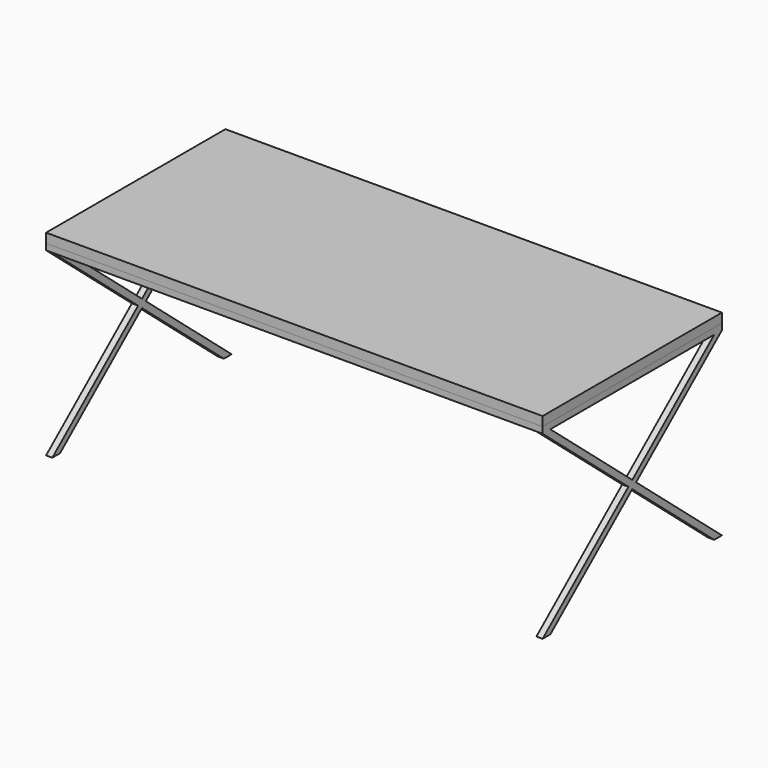
from build123d import *

# Parameters (mm, degrees)
F1_DEPTH = 25.4
F5_W     = 2025.65
F5_H     = 914.4
F6_DEPTH = 38.1
F7_W     = 1974.85
F7_H     = 25.4
F7_W_2   = 2000.25
F8_DEPTH = 25.4


# Not quite as in the source:
# - a feature of the source that left no trace in its solid (it failed there, or was rolled back) is left out
# - a pattern or mirror of a feature is missing from the dataset's text; its kind, count and spacing are read off the source's solid


with BuildPart() as f1:
    # F0 (on Right) → F1 (new body)
    with BuildSketch(Plane.YZ):
        Polygon((-417.7607692471, 368.3), (-457.2, 368.3), (-19.7196153764, 0), (0, 16.6012799623), align=None)
        Polygon((-457.2, 393.7), (-457.2, 368.3), (-417.7607692471, 368.3), (417.7607692471, 368.3), (457.2, 368.3), (457.2, 393.7), align=None)
        Polygon((0, 16.6012799623), (-19.7196153764, 0), (0, -16.6012799623), (19.7196153764, 0), align=None)
        Polygon((0, -16.6012799623), (-19.7196153764, 0), (-457.2, -368.3), (-417.7607692471, -368.3), align=None)
        Polygon((19.7196153764, 0), (0, -16.6012799623), (417.7607692471, -368.3), (457.2, -368.3), align=None)
        Polygon((417.7607692471, 368.3), (0, 16.6012799623), (19.7196153764, 0), (457.2, 368.3), align=None)
    extrude(amount=-F1_DEPTH)


with BuildPart() as f1_copies_1:
    # F1_copies: instance of F1
    add(f1.part.mirror(Plane(origin=(-1012.825, 0, 0), x_dir=(0, 0, -1), z_dir=(-1, 0, 0))))


with BuildPart() as f6:
    # F5 (on face) → F6 (new body)
    with BuildSketch(Plane.XY.offset(393.7)):
        with Locations((-1012.825, 0)):
            Rectangle(F5_W, F5_H)
    extrude(amount=F6_DEPTH)


with BuildPart() as f1_1:
    add(f1.part)

    add(f1_copies_1.part)  # F8 merges F1_copies_1
    # F7 (on face) → F8 (join)
    with BuildSketch(Plane.XY.offset(393.7)):
        with Locations((-1012.825, 444.5)):
            Rectangle(F7_W, F7_H)
        with Locations((-1025.525, -444.5)):
            Rectangle(F7_W_2, F7_H)
    extrude(amount=-F8_DEPTH)


solid = Compound([f6.part, f1_1.part])
